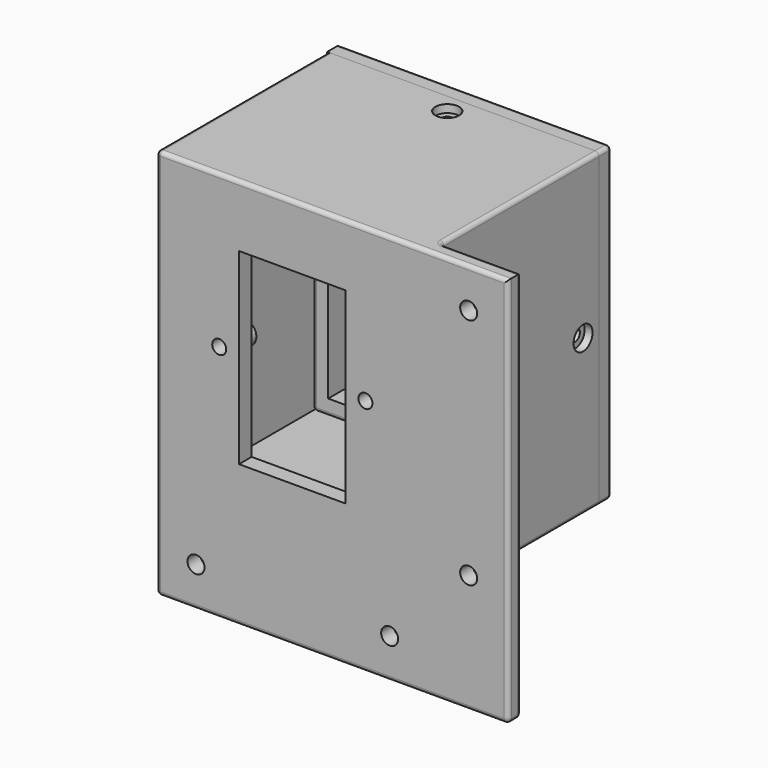
from build123d import *

# Parameters (mm, degrees)
F0_R      = 2.15
F0_R_2    = 3
F0_W      = 27
F0_H      = 47.5
F0_R_3    = 1.77
F1_DEPTH  = 4
F2_DEPTH  = 8
F3_W      = 68.75
F3_H      = 78.75
F3_W_2    = 60.75
F3_H_2    = 70.75
F4_DEPTH  = 50
F5_W      = 68.75
F5_H      = 78.75
F6_DEPTH  = 4
F7_W      = 52.25
F7_H      = 62.25
F8_DEPTH  = 10
F9_R      = 1
F10_R     = 1.5
F11_DEPTH = 25
F10_R_2   = 3
F12_DEPTH = 2
F13_R     = 1.5
F14_DEPTH = 89.001
F13_R_2   = 3
F15_DEPTH = 2
F16_R     = 3
F16_R_2   = 1.5
F17_DEPTH = 2
F18_R     = 1
F18_2_R   = 1


with BuildPart() as f1:
    # F0 (on Front) → F1 (new body)
    with BuildSketch(Plane.XZ):
        Polygon((-89, 0), (0, 0), (0, 99), (-20.25, 99), (-89, 99), align=None)
        with Locations((-79, 10)):
            Circle(F0_R, mode=Mode.SUBTRACT)
        with Locations((-30, 10)):
            Circle(F0_R, mode=Mode.SUBTRACT)
        with Locations((-10, 30)):
            Circle(F0_R, mode=Mode.SUBTRACT)
        with Locations((-73.125, 60.375)):
            Circle(F0_R_2, mode=Mode.SUBTRACT)
        with Locations((-54.625, 59.625)):
            Rectangle(F0_W, F0_H, mode=Mode.SUBTRACT)
        with Locations((-36.125, 60.375)):
            Circle(F0_R_2, mode=Mode.SUBTRACT)
        with Locations((-10, 89)):
            Circle(F0_R, mode=Mode.SUBTRACT)
        with Locations((-73.125, 60.375)):
            Circle(F0_R_2)
        with Locations((-73.125, 60.375)):
            Circle(F0_R_3, mode=Mode.SUBTRACT)
        with Locations((-36.125, 60.375)):
            Circle(F0_R_2)
        with Locations((-36.125, 60.375)):
            Circle(F0_R_3, mode=Mode.SUBTRACT)
    extrude(amount=-F1_DEPTH)

    # F0 (on Front) → F2 (join)
    with BuildSketch(Plane.XZ):
        with Locations((-73.125, 60.375)):
            Circle(F0_R_2)
        with Locations((-73.125, 60.375)):
            Circle(F0_R_3, mode=Mode.SUBTRACT)
        with Locations((-36.125, 60.375)):
            Circle(F0_R_2)
        with Locations((-36.125, 60.375)):
            Circle(F0_R_3, mode=Mode.SUBTRACT)
    extrude(amount=-F2_DEPTH)

    # F3 (on face) → F4 (join)
    with BuildSketch(Plane(origin=(0, 4, 0), x_dir=(-1, 0, 0), z_dir=(0, 1, 0))):
        with Locations((54.625, 59.625)):
            Rectangle(F3_W, F3_H)
        with Locations((54.625, 59.625)):
            Rectangle(F3_W_2, F3_H_2, mode=Mode.SUBTRACT)
    extrude(amount=F4_DEPTH)


with BuildPart() as f6:
    # F5 (on face) → F6 (new body)
    with BuildSketch(Plane(origin=(0, 54, 0), x_dir=(-1, 0, 0), z_dir=(0, 1, 0))):
        with Locations((54.625, 59.625)):
            Rectangle(F5_W, F5_H)
    extrude(amount=F6_DEPTH)

    # F7 (on face) → F8 (join)
    with BuildSketch(Plane.XZ.offset(-54)):
        Polygon((-80.75, 94.75), (-84.75, 94.75), (-84.75, 24.5), (-80.75, 24.5), (-28.5, 24.5), (-24.5, 24.5), (-24.5, 94.75), (-28.5, 94.75), align=None)
        with Locations((-54.625, 59.625)):
            Rectangle(F7_W, F7_H, mode=Mode.SUBTRACT)
    extrude(amount=F8_DEPTH)

    # F9
    f9_edges = [f6.edges().sort_by_distance(p)[0] for p in [
        (-54.625, 44, 94.75),
        (-84.75, 44, 59.625),
        (-24.5, 44, 59.625),
        (-54.625, 44, 24.5),
        (-84.75, 49, 94.75),
        (-84.75, 49, 24.5),
        (-24.5, 49, 24.5),
        (-24.5, 49, 94.75),
    ]]
    fillet(f9_edges, radius=F9_R)


with BuildPart() as f11_tool:
    # F10 (on face) → F11 (new body)
    with BuildSketch(Plane.XY.offset(99)):
        with Locations((-54.625, 49)):
            Circle(F10_R)
    extrude(amount=-F11_DEPTH)


with BuildPart() as f1_1:
    add(f1.part)

    # F11: cut by f11_tool
    add(f11_tool.part, mode=Mode.SUBTRACT)

    # F10 (on face) → F12 (cut)
    with BuildSketch(Plane.XY.offset(99)):
        with Locations((-54.625, 49)):
            Circle(F10_R_2)
        with Locations((-54.625, 49)):
            Circle(F10_R, mode=Mode.SUBTRACT)
    extrude(amount=-F12_DEPTH, mode=Mode.SUBTRACT)


with BuildPart() as f6_1:
    add(f6.part)

    # F11: cut by f11_tool
    add(f11_tool.part, mode=Mode.SUBTRACT)


with BuildPart() as f14_tool:
    # F13 (on face) → F14 (new body, through all)
    with BuildSketch(Plane(origin=(-89, 0, 0), x_dir=(0, -1, 0), z_dir=(-1, 0, 0))):
        with Locations((-49, 59.625)):
            Circle(F13_R)
    extrude(amount=-F14_DEPTH)


with BuildPart() as f1_2:
    add(f1_1.part)

    # F14: cut by f14_tool
    add(f14_tool.part, mode=Mode.SUBTRACT)

    # F13 (on face) → F15 (cut)
    with BuildSketch(Plane(origin=(-89, 0, 0), x_dir=(0, -1, 0), z_dir=(-1, 0, 0))):
        with Locations((-49, 59.625)):
            Circle(F13_R_2)
        with Locations((-49, 59.625)):
            Circle(F13_R, mode=Mode.SUBTRACT)
    extrude(amount=-F15_DEPTH, mode=Mode.SUBTRACT)

    # F16 (on face) → F17 (cut)
    with BuildSketch(Plane.YZ.offset(-20.25)):
        with Locations((49, 59.625)):
            Circle(F16_R)
        with Locations((49, 59.625)):
            Circle(F16_R_2, mode=Mode.SUBTRACT)
    extrude(amount=-F17_DEPTH, mode=Mode.SUBTRACT)

    # F18
    f18_edges = [f1_2.edges().sort_by_distance(p)[0] for p in [
        (0, 2, 0),
        (0, 0, 49.5),
        (-44.5, 0, 0),
        (-89, 0, 49.5),
        (-44.5, 0, 99),
        (-89, 2, 0),
        (-89, 4, 10.125),
        (-89, 27, 99),
        (-20.25, 4, 59.625),
        (-20.25, 29, 20.25),
        (-44.5, 4, 0),
        (0, 4, 49.5),
        (-10.125, 4, 99),
        (-54.625, 4, 20.25),
        (-20.25, 29, 99),
        (-89, 29, 20.25),
    ]]
    fillet(f18_edges, radius=F18_R)


with BuildPart() as f6_2:
    add(f6_1.part)

    # F14: cut by f14_tool
    add(f14_tool.part, mode=Mode.SUBTRACT)

    # F18#2
    f18_2_edges = [f6_2.edges().sort_by_distance(p)[0] for p in [
        (-54.625, 58, 99),
        (-20.25, 56, 99),
        (-20.25, 58, 59.625),
        (-20.25, 56, 20.25),
        (-54.625, 58, 20.25),
        (-89, 56, 20.25),
        (-89, 58, 59.625),
    ]]
    fillet(f18_2_edges, radius=F18_2_R)


solid = Compound([f1_2.part, f6_2.part])
